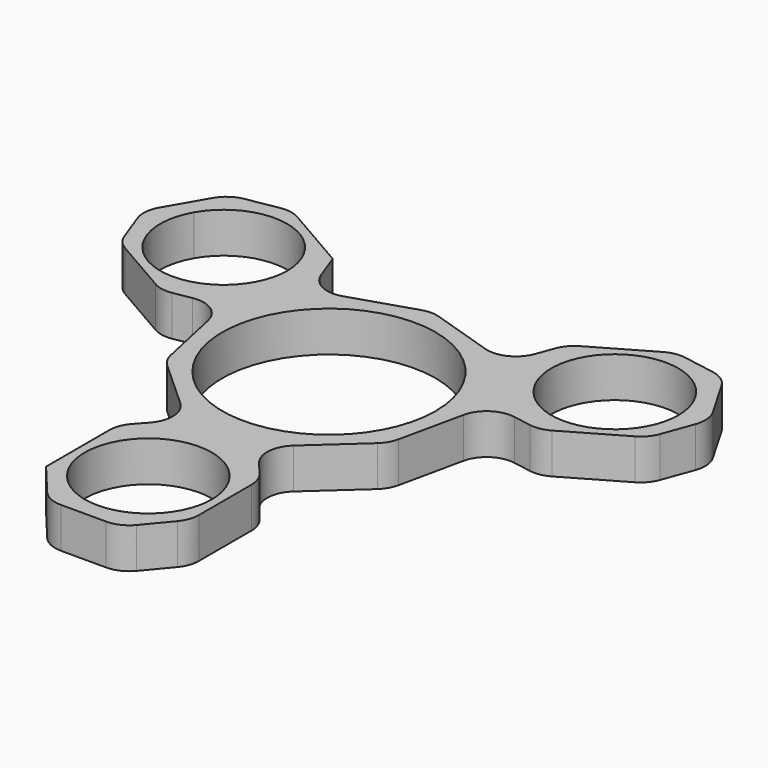
from build123d import *

# Parameters (mm, degrees)
F1_DEPTH  = 7
F3_R      = 18.475
F4_DEPTH  = 25
F5_W      = 25
F5_H      = 7
F6_DEPTH  = 30
F7_W      = 25
F7_H      = 7
F8_DEPTH  = 30
F9_W      = 25
F9_H      = 7
F10_DEPTH = 30
F12_DEPTH = 25
F14_DEPTH = 25
F16_DEPTH = 25
F17_R     = 5


with BuildPart() as f1:
    # F0 (on Top) → F1 (new body)
    with BuildSketch(Plane.XY):
        Polygon((-20, 34.6410161514), (0, 23.0940107676), (0, 69.2820323028), align=None)
        Polygon((0, 23.0940107676), (20, 34.6410161514), (0, 69.2820323028), align=None)
        Polygon((0, 23.0940107676), (40, 0), (20, 34.6410161514), align=None)
        Polygon((0, 0), (40, 0), (0, 23.0940107676), align=None)
        Polygon((-40, 0), (0, 0), (0, 23.0940107676), align=None)
        Polygon((-40, 0), (0, 23.0940107676), (-20, 34.6410161514), align=None)
    extrude(amount=F1_DEPTH)


with BuildPart() as f1_1:
    # F2: moved
    add(f1.part.moved(Location((0, -23.09401, 0))))

    # F3 (on face) → F4 (cut)
    with BuildSketch(Plane.XY.offset(7)):
        Circle(F3_R)
    extrude(amount=-F4_DEPTH, mode=Mode.SUBTRACT)

    # F5 (on face) → F6 (join)
    with BuildSketch(Plane.XZ.offset(23.09401)):
        with Locations((0, 3.5)):
            Rectangle(F5_W, F5_H)
    extrude(amount=F6_DEPTH)

    # F7 (on face) → F8 (join)
    with BuildSketch(Plane(origin=(20.0000003324, 11.5470055757, 0), x_dir=(-0.5, 0.8660254038, 0), z_dir=(0.8660254038, 0.5, 0))):
        with Locations((6.647e-07, 3.5)):
            Rectangle(F7_W, F7_H)
    extrude(amount=F8_DEPTH)

    # F9 (on face) → F10 (join)
    with BuildSketch(Plane(origin=(-20.0000003324, 11.5470055757, 0), x_dir=(-0.5, -0.8660254038, 0), z_dir=(-0.8660254038, 0.5, 0))):
        with Locations((0, 3.5)):
            Rectangle(F9_W, F9_H)
    extrude(amount=F10_DEPTH)

    # F11 (on face) → F12 (cut)
    with BuildSketch(Plane.XY.offset(7)):
        Polygon((0, 46.1880223028), (-13.7500003324, 22.372323123), (13.75, 22.3723236987), align=None)
        Polygon((26.25, 0.7216886041), (12.5, -23.09401), (40, -23.09401), align=None)
        Polygon((-12.5, -23.09401), (-26.2500003324, 0.7216880284), (-40, -23.09401), align=None)
    extrude(amount=-F12_DEPTH, mode=Mode.SUBTRACT)

    # F13 (on face) → F14 (cut)
    with BuildSketch(Plane.XY.offset(7)):
        with BuildLine():
            ThreePointArc((-22.8564067929, 19.5470055757), (-31.0093972968, 30.1721896649), (-43.3826862346, 25.0470055757))
            ThreePointArc((-43.3826862346, 25.0470055757), (-36.7034162891, 8.9218214865), (-22.8564067929, 19.5470055757))
        make_face()
        with BuildLine():
            ThreePointArc((44.8564064606, 19.5470061514), (44.4815905497, 22.3940156475), (43.3826859022, 25.0470061514))
            ThreePointArc((43.3826859022, 25.0470061514), (23.2312223714, 16.6999966552), (44.8564064606, 19.5470061514))
        make_face()
        with BuildLine():
            ThreePointArc((11, -39.09401), (-7.7781745931, -31.3158354069), (0, -50.09401))
            ThreePointArc((0, -50.09401), (7.7781745931, -46.8721845931), (11, -39.09401))
        make_face()
    extrude(amount=-F14_DEPTH, mode=Mode.SUBTRACT)

    # F15 (on face) → F16 (cut)
    with BuildSketch(Plane.XY.offset(7)):
        Polygon((-20.2451908608, 26.122323123), (-16.8750003324, 16.9596643493), (-13.7500003324, 22.372323123), align=None)
        Polygon((-13.7500003324, 22.372323123), (-16.8750003324, 16.9596643493), (-1.662e-07, 22.3723234108), align=None)
        Polygon((13.75, 22.3723236987), (-1.662e-07, 22.3723234108), (16.875, 16.959664925), align=None)
        Polygon((13.75, 22.3723236987), (16.875, 16.959664925), (20.2451905284, 26.1223236987), align=None)
        Polygon((32.7451905284, 4.4716886041), (23.125, 6.1343473777), (26.25, 0.7216886041), align=None)
        Polygon((23.125, 6.1343473777), (19.375, -11.186160698), (26.25, 0.7216886041), align=None)
        Polygon((19.375, -11.186160698), (6.25, -23.09401), (12.5, -23.09401), align=None)
        Polygon((12.5, -23.09401), (6.25, -23.09401), (12.5, -30.59401), align=None)
        Polygon((-12.5, -29.9828486929), (-6.25, -23.09401), (-12.5, -23.09401), align=None)
        Polygon((-6.25, -23.09401), (-19.3750001662, -11.1861609858), (-12.5, -23.09401), align=None)
        Polygon((-23.1250003324, 6.134346802), (-26.2500003324, 0.7216880284), (-19.3750001662, -11.1861609858), align=None)
        Polygon((-32.7451908608, 4.4716880284), (-26.2500003324, 0.7216880284), (-23.1250003324, 6.134346802), align=None)
        Polygon((-52.2307624459, 15.7216880284), (-45.7355719175, 11.9716880284), (-49.1057624459, 21.134346802), align=None)
        Polygon((-42.8557624459, 31.9596643493), (-33.2355719175, 33.622323123), (-39.7307624459, 37.372323123), align=None)
        Polygon((39.7307621135, 37.3723236987), (33.2355715851, 33.6223236987), (42.8557621135, 31.959664925), align=None)
        Polygon((49.1057621135, 21.1343473777), (45.7355715851, 11.9716886041), (52.2307621135, 15.7216886041), align=None)
        Polygon((12.5, -53.09401), (12.5, -45.59401), (6.25, -53.09401), align=None)
        Polygon((-6.25, -53.09401), (-12.5, -45.59401), (-12.5, -53.09401), align=None)
    extrude(amount=-F16_DEPTH, mode=Mode.SUBTRACT)

    # F17
    f17_edges = [f1_1.edges().sort_by_distance(p)[0] for p in [
        (6.25, -53.09401, 3.5),
        (12.5, -45.59401, 3.5),
        (12.5, -30.59401, 3.5),
        (-6.25, -53.09401, 3.5),
        (23.125, 6.134347, 3.5),
        (32.745191, 4.471689, 3.5),
        (45.735572, 11.971689, 3.5),
        (6.25, -23.09401, 3.5),
        (49.105762, 21.134347, 3.5),
        (42.855762, 31.959665, 3.5),
        (33.235572, 33.622324, 3.5),
        (20.245191, 26.122324, 3.5),
        (-33.235572, 33.622323, 3.5),
        (-12.5, -29.982849, 3.5),
        (-42.855762, 31.959664, 3.5),
        (-49.105762, 21.134347, 3.5),
        (-16.875, 16.959664, 3.5),
        (-23.125, 6.134347, 3.5),
        (-32.745191, 4.471688, 3.5),
        (-45.735572, 11.971688, 3.5),
        (-6.25, -23.09401, 3.5),
        (-19.375, -11.186161, 3.5),
        (0, 22.372323, 3.5),
        (16.875, 16.959665, 3.5),
        (19.375, -11.186161, 3.5),
    ]]
    fillet(f17_edges, radius=F17_R)


solid = f1_1.part
